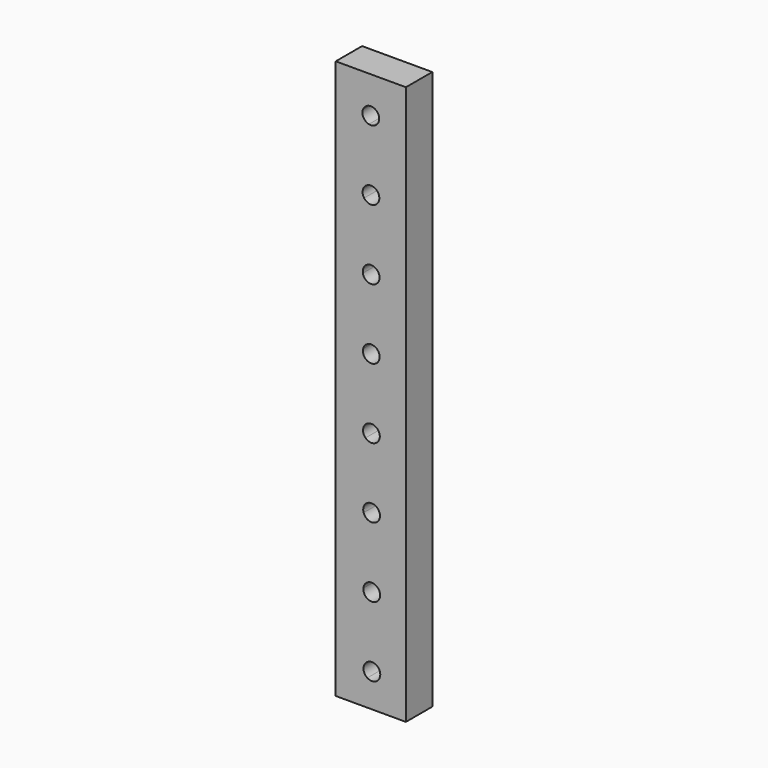
from build123d import *

# Parameters (mm, degrees)
F0_W     = 16.08
F0_H     = 2.6018508029
F1_DEPTH = 7.55


# Not quite as in the source:
# - the program builds the solid bodies; features that only make, move or delete a surface that nothing else refers to are left out


with BuildPart() as f1:
    # F0 (on Front) → F1 (new body)
    with BuildSketch(Plane.XZ):
        with Locations((-24.6192478486, 61.1047763503)):
            Rectangle(F0_W, F0_H)
        with BuildLine():
            Line((-16.5792478486, 59.8038509488), (-32.6592478486, 59.8038509488))
            Line((-32.6592478486, 59.8038509488), (-32.6592478486, 57.2638509407))
            Line((-32.6592478486, 57.2638509407), (-32.6592478486, 54.7238509326))
            Line((-32.6592478486, 54.7238509326), (-26.4178277978, 54.7238509326))
            ThreePointArc((-26.4178277978, 54.7238509326), (-24.6192478486, 55.9719058704), (-22.8206678995, 54.7238509326))
            ThreePointArc((-22.8206678995, 54.7238509326), (-22.7298466866, 54.3933194742), (-22.6992478486, 54.0519058704))
            ThreePointArc((-22.6992478486, 54.0519058704), (-23.1129129196, 52.8613786421), (-24.1756593919, 52.1838509245))
            ThreePointArc((-24.1756593919, 52.1838509245), (-24.6192478486, 52.1319058704), (-25.0628363054, 52.1838509245))
            Line((-25.0628363054, 52.1838509245), (-32.6592478486, 52.1838509245))
            Line((-32.6592478486, 52.1838509245), (-32.6592478486, 49.6438509164))
            Line((-32.6592478486, 49.6438509164), (-32.6592478486, 47.1038509083))
            Line((-32.6592478486, 47.1038509083), (-32.6592478486, 44.5638509002))
            Line((-32.6592478486, 44.5638509002), (-32.6592478486, 42.0238508921))
            Line((-32.6592478486, 42.0238508921), (-32.6592478486, 39.483850884))
            Line((-32.6592478486, 39.483850884), (-25.86093695, 39.483850884))
            ThreePointArc((-25.86093695, 39.483850884), (-24.5840999414, 39.9699445923), (-23.3072629328, 39.483850884))
            ThreePointArc((-23.3072629328, 39.483850884), (-22.8322541924, 38.8357158514), (-22.6640999414, 38.0499445923))
            ThreePointArc((-22.6640999414, 38.0499445923), (-22.7538524855, 37.4697771596), (-23.0147189518, 36.9438508759))
            ThreePointArc((-23.0147189518, 36.9438508759), (-24.5840999414, 36.1299445923), (-26.1534809311, 36.9438508759))
            Line((-26.1534809311, 36.9438508759), (-32.6592478486, 36.9438508759))
            Line((-32.6592478486, 36.9438508759), (-32.6592478486, 34.4038508678))
            Line((-32.6592478486, 34.4038508678), (-32.6592478486, 31.8638508597))
            Line((-32.6592478486, 31.8638508597), (-32.6592478486, 29.3238508516))
            Line((-32.6592478486, 29.3238508516), (-32.6592478486, 26.7838508435))
            Line((-32.6592478486, 26.7838508435), (-32.6592478486, 24.2438508354))
            Line((-32.6592478486, 24.2438508354), (-32.6592478486, 21.7038508273))
            Line((-32.6592478486, 21.7038508273), (-32.6592478486, 19.1638508192))
            Line((-32.6592478486, 19.1638508192), (-32.6592478486, 16.623850811))
            Line((-32.6592478486, 16.623850811), (-32.6592478486, 14.0838508029))
            Line((-32.6592478486, 14.0838508029), (-32.6592478486, 11.5438507948))
            Line((-32.6592478486, 11.5438507948), (-32.6592478486, 9.0038507867))
            Line((-32.6592478486, 9.0038507867), (-32.6592478486, 6.4638507786))
            Line((-32.6592478486, 6.4638507786), (-32.6592478486, 3.9238507705))
            Line((-32.6592478486, 3.9238507705), (-32.6592478486, 1.3838507624))
            Line((-32.6592478486, 1.3838507624), (-32.6592478486, -1.1561492457))
            Line((-32.6592478486, -1.1561492457), (-32.6592478486, -3.6961492538))
            Line((-32.6592478486, -3.6961492538), (-32.6592478486, -6.2361492619))
            Line((-32.6592478486, -6.2361492619), (-32.6592478486, -8.77614927))
            Line((-32.6592478486, -8.77614927), (-25.9934154817, -8.77614927))
            ThreePointArc((-25.9934154817, -8.77614927), (-24.4786562199, -8.0359392423), (-22.9638969581, -8.77614927))
            ThreePointArc((-22.9638969581, -8.77614927), (-22.6627903407, -9.3322156588), (-22.5586562199, -9.9559392423))
            ThreePointArc((-22.5586562199, -9.9559392423), (-22.705503056, -10.6923683681), (-23.1235810713, -11.3161492781))
            ThreePointArc((-23.1235810713, -11.3161492781), (-24.4786562199, -11.8759392423), (-25.8337313686, -11.3161492781))
            Line((-25.8337313686, -11.3161492781), (-32.6592478486, -11.3161492781))
            Line((-32.6592478486, -11.3161492781), (-32.6592478486, -13.8561492862))
            Line((-32.6592478486, -13.8561492862), (-32.6592478486, -16.3961492943))
            Line((-32.6592478486, -16.3961492943), (-32.6592478486, -18.9361493024))
            Line((-32.6592478486, -18.9361493024), (-32.6592478486, -21.4761493105))
            Line((-32.6592478486, -21.4761493105), (-32.6592478486, -24.0161493186))
            Line((-32.6592478486, -24.0161493186), (-32.6592478486, -26.5561493267))
            Line((-32.6592478486, -26.5561493267), (-32.6592478486, -29.0961493348))
            Line((-32.6592478486, -29.0961493348), (-32.6592478486, -31.6361493429))
            Line((-32.6592478486, -31.6361493429), (-32.6592478486, -34.176149351))
            Line((-32.6592478486, -34.176149351), (-32.6592478486, -36.7161493591))
            Line((-32.6592478486, -36.7161493591), (-32.6592478486, -39.2561493672))
            Line((-32.6592478486, -39.2561493672), (-32.6592478486, -41.7961493753))
            Line((-32.6592478486, -41.7961493753), (-32.6592478486, -44.3361493834))
            Line((-32.6592478486, -44.3361493834), (-32.6592478486, -46.8761493915))
            Line((-32.6592478486, -46.8761493915), (-32.6592478486, -49.4161493996))
            Line((-32.6592478486, -49.4161493996), (-32.6592478486, -51.9561494077))
            Line((-32.6592478486, -51.9561494077), (-32.6592478486, -54.4961494159))
            Line((-32.6592478486, -54.4961494159), (-32.6592478486, -57.036149424))
            Line((-32.6592478486, -57.036149424), (-26.0553326749, -57.036149424))
            ThreePointArc((-26.0553326749, -57.036149424), (-24.3732124984, -56.0418230768), (-22.6910923218, -57.036149424))
            ThreePointArc((-22.6910923218, -57.036149424), (-22.5136331455, -57.4839479566), (-22.4532124984, -57.9618230768))
            ThreePointArc((-22.4532124984, -57.9618230768), (-22.6876790209, -58.8812668742), (-23.3338134322, -59.5761494321))
            ThreePointArc((-23.3338134322, -59.5761494321), (-24.3732124984, -59.8818230768), (-25.4126115646, -59.5761494321))
            Line((-25.4126115646, -59.5761494321), (-32.6592478486, -59.5761494321))
            Line((-32.6592478486, -59.5761494321), (-32.6592478486, -62.1161494402))
            Line((-32.6592478486, -62.1161494402), (-32.6592478486, -65.5842982483))
            Line((-32.6592478486, -65.5842982483), (-16.5792478486, -65.5842982483))
            Line((-16.5792478486, -65.5842982483), (-16.5792478486, 59.8038509488))
        make_face()
        with BuildLine():
            ThreePointArc((-22.4883604056, -41.9598617986), (-24.4902912462, -43.8781129129), (-26.3213680486, -41.7961493753))
            ThreePointArc((-26.3213680486, -41.7961493753), (-24.4083604056, -40.0398617986), (-22.4953527625, -41.7961493753))
            ThreePointArc((-22.4953527625, -41.7961493753), (-22.4901092913, -41.877930958), (-22.4883604056, -41.9598617986))
        make_face(mode=Mode.SUBTRACT)
        with BuildLine():
            ThreePointArc((-22.6190910453, -26.5561493267), (-24.4435083127, -27.8779005205), (-26.2679255802, -26.5561493267))
            ThreePointArc((-26.2679255802, -26.5561493267), (-24.7464264918, -24.0619467824), (-22.5235083127, -25.9579005205))
            ThreePointArc((-22.5235083127, -25.9579005205), (-22.5475545747, -26.2608186996), (-22.6190910453, -26.5561493267))
        make_face(mode=Mode.SUBTRACT)
        with BuildLine():
            ThreePointArc((-22.5938041271, 6.0460220359), (-24.7239815843, 4.1375604994), (-26.3877889567, 6.4638507786))
            ThreePointArc((-26.3877889567, 6.4638507786), (-24.5138041271, 7.9660220359), (-22.6398192974, 6.4638507786))
            ThreePointArc((-22.6398192974, 6.4638507786), (-22.6053425905, 6.2561994932), (-22.5938041271, 6.0460220359))
        make_face(mode=Mode.SUBTRACT)
        with BuildLine():
            ThreePointArc((-22.6600441933, 21.7038508273), (-24.5489520343, 20.1279833141), (-26.4378598752, 21.7038508273))
            ThreePointArc((-26.4378598752, 21.7038508273), (-24.7217191397, 23.9601944759), (-22.6289520343, 22.0479833141))
            ThreePointArc((-22.6289520343, 22.0479833141), (-22.6367408725, 21.8752162087), (-22.6600441933, 21.7038508273))
        make_face(mode=Mode.SUBTRACT)
        with BuildLine():
            Line((-26.4178277978, 54.7238509326), (-32.6592478486, 54.7238509326))
            Line((-32.6592478486, 54.7238509326), (-32.6592478486, 52.1838509245))
            Line((-32.6592478486, 52.1838509245), (-25.0628363054, 52.1838509245))
            ThreePointArc((-25.0628363054, 52.1838509245), (-26.3132755345, 53.1482078016), (-26.4178277978, 54.7238509326))
        make_face()
        with BuildLine():
            Line((-32.6592478486, -57.036149424), (-32.6592478486, -59.5761494321))
            Line((-32.6592478486, -59.5761494321), (-25.4126115646, -59.5761494321))
            ThreePointArc((-25.4126115646, -59.5761494321), (-26.2345471694, -58.4328148417), (-26.0553326749, -57.036149424))
            Line((-26.0553326749, -57.036149424), (-32.6592478486, -57.036149424))
        make_face()
        with BuildLine():
            Line((-25.86093695, 39.483850884), (-32.6592478486, 39.483850884))
            Line((-32.6592478486, 39.483850884), (-32.6592478486, 36.9438508759))
            Line((-32.6592478486, 36.9438508759), (-26.1534809311, 36.9438508759))
            ThreePointArc((-26.1534809311, 36.9438508759), (-26.4914906287, 38.2696279242), (-25.86093695, 39.483850884))
        make_face()
        with BuildLine():
            Line((-32.6592478486, -8.77614927), (-32.6592478486, -11.3161492781))
            Line((-32.6592478486, -11.3161492781), (-25.8337313686, -11.3161492781))
            ThreePointArc((-25.8337313686, -11.3161492781), (-26.394873169, -10.0764075113), (-25.9934154817, -8.77614927))
            Line((-25.9934154817, -8.77614927), (-32.6592478486, -8.77614927))
        make_face()
    extrude(amount=F1_DEPTH)


solid = f1.part
